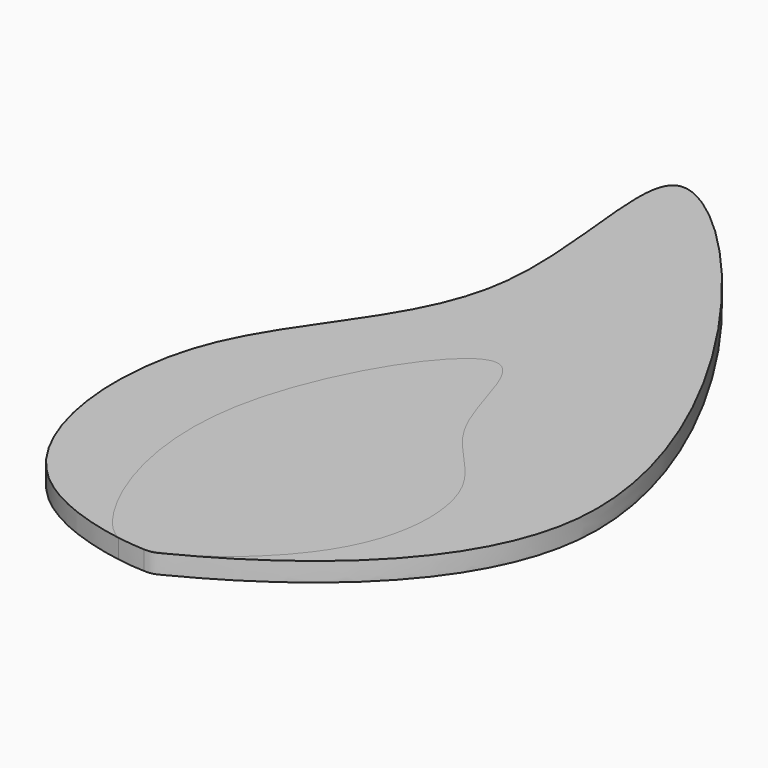
from build123d import *

# Parameters (mm, degrees)
F1_DEPTH = 2.54
F2_DEPTH = 2.54


with BuildPart() as f1:
    # F0 (on Top) → F1 (new body)
    with BuildSketch(Plane.XY):
        with BuildLine():
            add(Edge.make_bspline(
                [(-6.2375405564, -46.2178631648), (-7.307276746, -45.6717733468), (-12.0675351695, -40.9823170252), (-21.5930596382, -16.3432652524), (1.8568971434, 19.4274825185), (4.5509972625, -6.0200594515), (16.8123086502, -13.1301159921), (17.2421105498, -33.9336012457), (2.4005706068, -45.5843690827), (-2.4912711233, -46.6105885752)],
                knots=[0.046178655, 0.046178655, 0.046178655, 0.046178655, 0.0915716184, 0.2713991814, 0.4513125898, 0.5777389143, 0.7028550953, 0.8448074849, 1, 1, 1, 1], degree=3))
            add(Edge.make_bspline(
                [(-2.4912711233, -46.6105885752), (-1.4199750088, -46.6396392568), (-0.345071475, -46.0389480469), (55.9237069542, -16.8608488775), (-23.0338192489, 78.286040227), (-3.66143577, 17.438695129), (-32.2132933669, -2.6742848508), (-27.6051608315, -40.6562967051), (-10.4143382247, -45.5341023771), (-6.2375405564, -46.2178631648)],
                knots=[0, 0, 0, 0, 0.0419852951, 0.2155713527, 0.4415540311, 0.5812706992, 0.7339643286, 0.8846807143, 0.9679448078, 0.9679448078, 0.9679448078, 0.9679448078], degree=3))
        make_face()
    extrude(amount=F1_DEPTH)


with BuildPart() as f2:
    # F0 (on Top) → F2 (new body)
    with BuildSketch(Plane.XY):
        with BuildLine():
            add(Edge.make_bspline(
                [(-6.2375405564, -46.2178631648), (-4.6295478885, -46.4810988829), (-3.3091908909, -46.5884087815), (-2.4912711233, -46.6105885752)],
                knots=[0.9679448078, 0.9679448078, 0.9679448078, 0.9679448078, 1, 1, 1, 1], degree=3))
            add(Edge.make_bspline(
                [(-6.2375405564, -46.2178631648), (-7.307276746, -45.6717733468), (-12.0675351695, -40.9823170252), (-21.5930596382, -16.3432652524), (1.8568971434, 19.4274825185), (4.5509972625, -6.0200594515), (16.8123086502, -13.1301159921), (17.2421105498, -33.9336012457), (2.4005706068, -45.5843690827), (-2.4912711233, -46.6105885752)],
                knots=[0.046178655, 0.046178655, 0.046178655, 0.046178655, 0.0915716184, 0.2713991814, 0.4513125898, 0.5777389143, 0.7028550953, 0.8448074849, 1, 1, 1, 1], degree=3))
        make_face()
    extrude(amount=F2_DEPTH)


solid = Compound([f1.part, f2.part])
